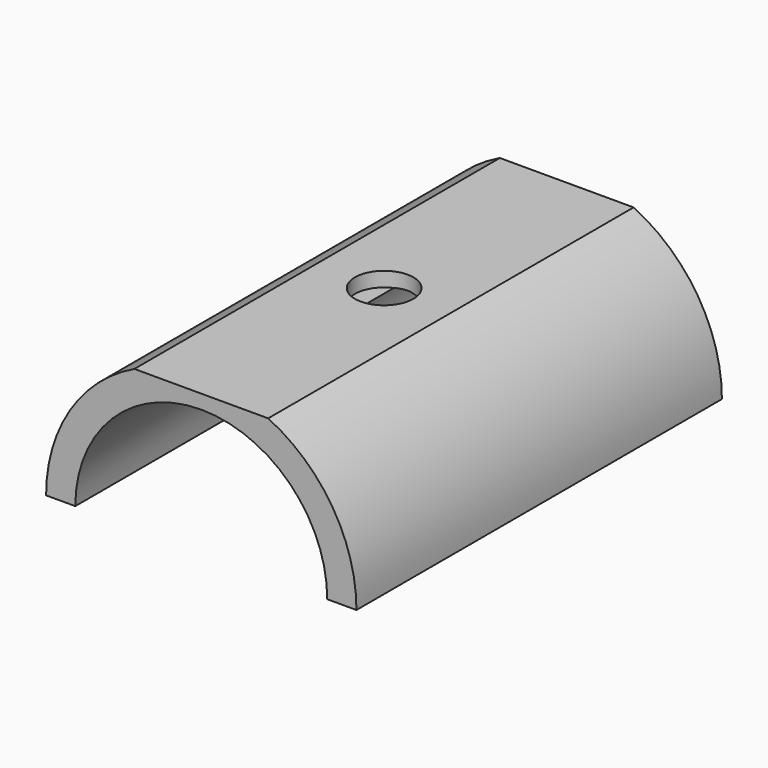
from build123d import *

# Parameters (mm, degrees)
F1_DEPTH = 125.1
F2_W     = 44
F2_H     = 7.301
F3_DEPTH = 125.1
F4_R     = 8
F5_DEPTH = 4


with BuildPart() as f1:
    # F0 (on Front) → F1 (new body)
    with BuildSketch(Plane.XZ):
        with BuildLine():
            ThreePointArc((-34.5, 0), (0, 34.5), (34.5, 0))
            Line((34.5, 0), (42.5, 0))
            ThreePointArc((42.5, 0), (0, 42.5), (-42.5, 0))
            Line((-42.5, 0), (-34.5, 0))
        make_face()
    extrude(amount=F1_DEPTH)

    # F2 (on Front) → F3 (cut)
    with BuildSketch(Plane.XZ):
        with Locations((0, 42)):
            Rectangle(F2_W, F2_H)
    extrude(amount=F3_DEPTH, mode=Mode.SUBTRACT)

    # F4 (on face) → F5 (cut)
    with BuildSketch(Plane.XY.offset(38.3495)):
        with Locations((0, -62.5)):
            Circle(F4_R)
    extrude(amount=-F5_DEPTH, mode=Mode.SUBTRACT)


solid = f1.part
